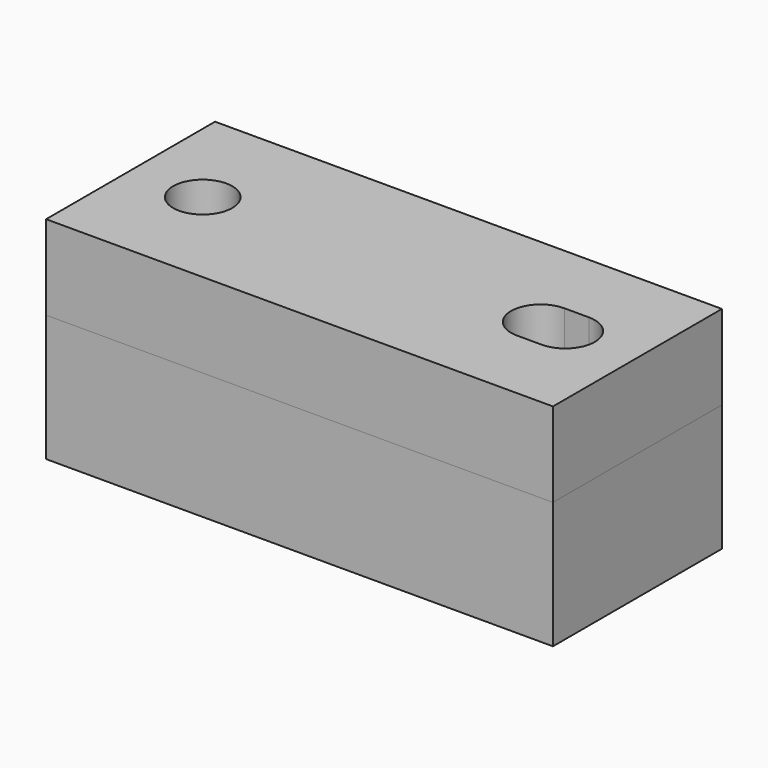
from build123d import *

# Parameters (mm, degrees)
F0_W      = 60
F0_H      = 15
F1_DEPTH  = 12.5
F4_W      = 1
F4_H      = 12
F6_W      = 60
F6_H      = 10
F7_DEPTH  = 12.5
F8_W      = 3.5002815183
F8_H      = 10
F11_DEPTH = 25
F14_W     = 1
F14_H     = 12


# Not quite as in the source:
# - a pattern or mirror of a feature is missing from the dataset's text; its kind, count and spacing are read off the source's solid


with BuildPart() as f1:
    # F0 (on Front) → F1 (new body, symmetric)
    with BuildSketch(Plane.XZ):
        with Locations((0, -7.5)):
            Rectangle(F0_W, F0_H)
    extrude(amount=F1_DEPTH, both=True)

    # F2 (on Front) → F3 (revolve, cut)
    with BuildSketch(Plane.XZ):
        Polygon((-21.9591817715, -12.4931969619), (-18.7036573682, -13.778055791), (-22, 6), (-24.9591817715, 5.5068030381), align=None)
    f3 = revolve(axis=Axis((-20.3518286841, 0, -3.8890278955), (-0.1643989873, 0, 0.9863939238)), mode=Mode.SUBTRACT)

    # F3_copies: F3 across plane
    add(f3.mirror(Plane(origin=(0, 0, 0), x_dir=(0, 0, 1), z_dir=(1, 0, 0))), mode=Mode.SUBTRACT)


with BuildPart() as f5:
    # F4 (on Front) → F5 (revolve)
    with BuildSketch(Plane.XZ):
        with Locations((-20.5, -6)):
            Rectangle(F4_W, F4_H)
    revolve(axis=Axis((-20, 0, -6), (0, 0, -1)))


with BuildPart() as f7:
    # F6 (on Front) → F7 (new body, symmetric)
    with BuildSketch(Plane.XZ):
        with Locations((0, 5)):
            Rectangle(F6_W, F6_H)
    extrude(amount=F7_DEPTH, both=True)

    # F8 (on Front) → F9 (revolve, cut)
    with BuildSketch(Plane.XZ):
        with Locations((-23.2090410123, 5)):
            Rectangle(F8_W, F8_H)
    revolve(axis=Axis((-21.4589002532, 0, 5), (0, 0, 1)), mode=Mode.SUBTRACT)

    # F10 (on face) → F11 (cut)
    with BuildSketch(Plane.XY.offset(10)):
        with BuildLine():
            Line((21.4589002532, 3.5002815183), (18.5410997468, 3.5002815183))
            ThreePointArc((18.5410997468, 3.5002815183), (15.0408182285, 0), (18.5410997468, -3.5002815183))
            Line((18.5410997468, -3.5002815183), (21.4589002532, -3.5002815183))
            ThreePointArc((21.4589002532, -3.5002815183), (24.9591817715, 0), (21.4589002532, 3.5002815183))
        make_face()
    extrude(amount=-F11_DEPTH, mode=Mode.SUBTRACT)


with BuildPart() as f13:
    # F12 (on Front) → F13 (revolve)
    with BuildSketch(Plane.XZ):
        Polygon((-24.9591817715, 5.5068030381), (-22.3287979746, -10.2754997432), (-19.3696162031, -9.7823027813), (-22, 6), align=None)
    revolve(axis=Axis((-20.6848081016, 0, -1.8911513907), (0.1643989873, 0, -0.9863939238)))


with BuildPart() as f13_copies_1:
    # F13_copies: instance of F13
    add(f13.part.mirror(Plane(origin=(0, 0, 0), x_dir=(0, 0, 1), z_dir=(1, 0, 0))))


with BuildPart() as f13_1:
    add(f13.part)

    # F14 (on Front) → F15 (revolve, cut)
    with BuildSketch(Plane.XZ):
        with Locations((-20.5, -6)):
            Rectangle(F14_W, F14_H)
    revolve(axis=Axis((-20, 0, -6), (0, 0, 1)), mode=Mode.SUBTRACT)


solid = Compound([f1.part, f5.part, f7.part, f13_copies_1.part, f13_1.part])
